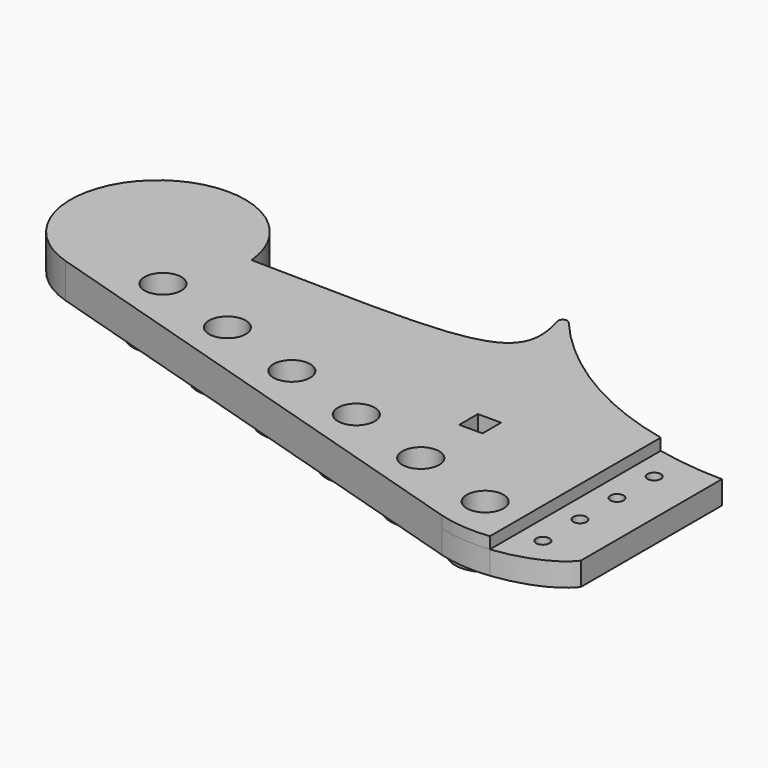
from build123d import *

# Parameters (mm, degrees)
F0_R      = 5.0419
F1_DEPTH  = 6.35
F2_DEPTH  = 9.525
F4_D      = 3.6576
F5_R      = 1.27
F8_W      = 6.35
F8_H      = 6.35
F9_DEPTH  = 9.5260001
F10_R     = 5.0419
F11_DEPTH = 3.175


with BuildPart() as f1:
    # F0 (on Top) → F1 (new body)
    with BuildSketch(Plane.XY):
        with BuildLine():
            Line((0, 0), (0, 24.13))
            ThreePointArc((0, 24.13), (-9.2620503813, 24.6926494565), (-18.415, 26.2176625565))
            Line((-18.415, 26.2176625565), (-18.415, -32.2023374435))
            add(Edge.make_bspline(
                [(-18.415, -32.2023374435), (-10.35310168, -31.3379440787), (-3.0120759205, -28.1461012273), (0, -24.13)],
                knots=[12.2106695442, 12.2106695442, 12.2106695442, 12.2106695442, 33.2224141479, 33.2224141479, 33.2224141479, 33.2224141479], degree=3))
            Line((0, -24.13), (0, 0))
        make_face()
        with BuildLine():
            Line((-18.415, -32.2023374435), (-18.415, 26.2176625565))
            ThreePointArc((-18.415, 26.2176625565), (-48.7549341061, 39.1874227389), (-72.2748938826, 62.3291118058))
            add(Edge.make_bspline(
                [(-137.9783539955, 35.7469866649), (-73.1067731977, 34.5293954015), (-59.7019699566, 33.2077455579), (-72.2748938826, 62.3291118058)],
                knots=[0, 0, 0, 0, 70.8770346997, 70.8770346997, 70.8770346997, 70.8770346997], degree=3))
            ThreePointArc((-137.9783539955, 35.7469866649), (-162.9147928474, 57.3381501066), (-185.674, 33.4629996115))
            ThreePointArc((-185.674, 33.4629996115), (-180.9856867862, 19.2452424177), (-168.7599080893, 10.6049162859))
            Line((-168.7599080893, 10.6049162859), (-32.4923986546, -31.0562422342))
            add(Edge.make_bspline(
                [(-32.4923986546, -31.0562422342), (-28.0285616621, -32.4209741599), (-23.1000548653, -32.7046670659), (-18.415, -32.2023374435)],
                knots=[0, 0, 0, 0, 12.2106695442, 12.2106695442, 12.2106695442, 12.2106695442], degree=3))
        make_face()
        with Locations((-99.2384759306, 1.0898536678)):
            Circle(F0_R, mode=Mode.SUBTRACT)
        with Locations((-122.5813012408, 8.226471557)):
            Circle(F0_R, mode=Mode.SUBTRACT)
        with Locations((-52.5528253102, -13.1833821107)):
            Circle(F0_R, mode=Mode.SUBTRACT)
        with Locations((-29.21, -20.32)):
            Circle(F0_R, mode=Mode.SUBTRACT)
        with Locations((-75.8956506204, -6.0467642215)):
            Circle(F0_R, mode=Mode.SUBTRACT)
        with Locations((-145.924126551, 15.3630894463)):
            Circle(F0_R, mode=Mode.SUBTRACT)
    extrude(amount=F1_DEPTH)

    # F0 (on Top) → F2 (join)
    with BuildSketch(Plane.XY):
        with BuildLine():
            Line((-18.415, -32.2023374435), (-18.415, 26.2176625565))
            ThreePointArc((-18.415, 26.2176625565), (-48.7549341061, 39.1874227389), (-72.2748938826, 62.3291118058))
            add(Edge.make_bspline(
                [(-137.9783539955, 35.7469866649), (-73.1067731977, 34.5293954015), (-59.7019699566, 33.2077455579), (-72.2748938826, 62.3291118058)],
                knots=[0, 0, 0, 0, 70.8770346997, 70.8770346997, 70.8770346997, 70.8770346997], degree=3))
            ThreePointArc((-137.9783539955, 35.7469866649), (-162.9147928474, 57.3381501066), (-185.674, 33.4629996115))
            ThreePointArc((-185.674, 33.4629996115), (-180.9856867862, 19.2452424177), (-168.7599080893, 10.6049162859))
            Line((-168.7599080893, 10.6049162859), (-32.4923986546, -31.0562422342))
            add(Edge.make_bspline(
                [(-32.4923986546, -31.0562422342), (-28.0285616621, -32.4209741599), (-23.1000548653, -32.7046670659), (-18.415, -32.2023374435)],
                knots=[0, 0, 0, 0, 12.2106695442, 12.2106695442, 12.2106695442, 12.2106695442], degree=3))
        make_face()
        with Locations((-99.2384759306, 1.0898536678)):
            Circle(F0_R, mode=Mode.SUBTRACT)
        with Locations((-122.5813012408, 8.226471557)):
            Circle(F0_R, mode=Mode.SUBTRACT)
        with Locations((-52.5528253102, -13.1833821107)):
            Circle(F0_R, mode=Mode.SUBTRACT)
        with Locations((-29.21, -20.32)):
            Circle(F0_R, mode=Mode.SUBTRACT)
        with Locations((-75.8956506204, -6.0467642215)):
            Circle(F0_R, mode=Mode.SUBTRACT)
        with Locations((-145.924126551, 15.3630894463)):
            Circle(F0_R, mode=Mode.SUBTRACT)
    extrude(amount=F2_DEPTH)

    # F4 (through all)
    with Locations(Plane.XY.offset(6.35)):
        with Locations((-12.065, 16.0576625565), (-12.065, 3.3576625565), (-12.065, -9.3423374435), (-12.065, -22.0423374435)):
            Hole(F4_D / 2)

    # F5
    f5_edges = [f1.edges().sort_by_distance(p)[0] for p in [
        (-72.274894, 62.329112, 3.175),
        (-72.274894, 62.329112, 7.9375),
    ]]
    fillet(f5_edges, radius=F5_R)

    # F8 (on Top) → F9 (cut, through all)
    with BuildSketch(Plane.XY):
        with Locations((-52.5528253102, 7.1366178893)):
            Rectangle(F8_W, F8_H)
    extrude(amount=F9_DEPTH, mode=Mode.SUBTRACT)

    # F10 (on face) → F11 (join)
    with BuildSketch(Plane(origin=(0, 0, 0), x_dir=(1, 0, 0), z_dir=(0, 0, -1))):
        with BuildLine():
            ThreePointArc((-29.21, 12.1031), (-23.3997742897, 14.5097742897), (-20.9931, 20.32))
            ThreePointArc((-20.9931, 20.32), (-29.21, 28.5369), (-37.4269, 20.32))
            ThreePointArc((-37.4269, 20.32), (-35.0202257103, 14.5097742897), (-29.21, 12.1031))
        make_face()
        with Locations((-29.21, 20.32)):
            Circle(F10_R, mode=Mode.SUBTRACT)
        with BuildLine():
            ThreePointArc((-29.21, 12.1031), (-35.0202257103, 14.5097742897), (-37.4269, 20.32))
            Line((-37.4269, 20.32), (-37.4269, 12.1031))
            Line((-37.4269, 12.1031), (-29.21, 12.1031))
        make_face()
        with BuildLine():
            ThreePointArc((-52.5528253102, 4.9664821107), (-58.3630510205, 7.3731564004), (-60.7697253102, 13.1833821107))
            Line((-60.7697253102, 13.1833821107), (-60.7697253102, 4.9664821107))
            Line((-60.7697253102, 4.9664821107), (-52.5528253102, 4.9664821107))
        make_face()
        with BuildLine():
            ThreePointArc((-44.3359253102, 13.1833821107), (-52.5528253102, 21.4002821107), (-60.7697253102, 13.1833821107))
            ThreePointArc((-60.7697253102, 13.1833821107), (-58.3630510205, 7.3731564004), (-52.5528253102, 4.9664821107))
            ThreePointArc((-52.5528253102, 4.9664821107), (-46.7425995999, 7.3731564004), (-44.3359253102, 13.1833821107))
        make_face()
        with Locations((-52.5528253102, 13.1833821107)):
            Circle(F10_R, mode=Mode.SUBTRACT)
        with BuildLine():
            ThreePointArc((-75.8956506204, -2.1701357785), (-81.7058763307, 0.2365385111), (-84.1125506204, 6.0467642215))
            Line((-84.1125506204, 6.0467642215), (-84.1125506204, -2.1701357785))
            Line((-84.1125506204, -2.1701357785), (-75.8956506204, -2.1701357785))
        make_face()
        with BuildLine():
            ThreePointArc((-67.6787506204, 6.0467642215), (-75.8956506204, 14.2636642215), (-84.1125506204, 6.0467642215))
            ThreePointArc((-84.1125506204, 6.0467642215), (-81.7058763307, 0.2365385111), (-75.8956506204, -2.1701357785))
            ThreePointArc((-75.8956506204, -2.1701357785), (-70.0854249101, 0.2365385111), (-67.6787506204, 6.0467642215))
        make_face()
        with Locations((-75.8956506204, 6.0467642215)):
            Circle(F10_R, mode=Mode.SUBTRACT)
        with BuildLine():
            ThreePointArc((-99.2384759306, -9.3067536678), (-105.0487016409, -6.9000793781), (-107.4553759306, -1.0898536678))
            Line((-107.4553759306, -1.0898536678), (-107.4553759306, -9.3067536678))
            Line((-107.4553759306, -9.3067536678), (-99.2384759306, -9.3067536678))
        make_face()
        with BuildLine():
            ThreePointArc((-91.0215759306, -1.0898536678), (-99.2384759306, 7.1270463322), (-107.4553759306, -1.0898536678))
            ThreePointArc((-107.4553759306, -1.0898536678), (-105.0487016409, -6.9000793781), (-99.2384759306, -9.3067536678))
            ThreePointArc((-99.2384759306, -9.3067536678), (-93.4282502203, -6.9000793781), (-91.0215759306, -1.0898536678))
        make_face()
        with Locations((-99.2384759306, -1.0898536678)):
            Circle(F10_R, mode=Mode.SUBTRACT)
        with BuildLine():
            ThreePointArc((-122.5813012408, -16.443371557), (-128.3915269511, -14.0366972674), (-130.7982012408, -8.226471557))
            Line((-130.7982012408, -8.226471557), (-130.7982012408, -16.443371557))
            Line((-130.7982012408, -16.443371557), (-122.5813012408, -16.443371557))
        make_face()
        with BuildLine():
            ThreePointArc((-114.3644012408, -8.226471557), (-122.5813012408, -0.009571557), (-130.7982012408, -8.226471557))
            ThreePointArc((-130.7982012408, -8.226471557), (-128.3915269511, -14.0366972674), (-122.5813012408, -16.443371557))
            ThreePointArc((-122.5813012408, -16.443371557), (-116.7710755305, -14.0366972674), (-114.3644012408, -8.226471557))
        make_face()
        with Locations((-122.5813012408, -8.226471557)):
            Circle(F10_R, mode=Mode.SUBTRACT)
        with BuildLine():
            ThreePointArc((-145.924126551, -23.5799894463), (-151.7343522614, -21.1733151566), (-154.141026551, -15.3630894463))
            Line((-154.141026551, -15.3630894463), (-154.141026551, -23.5799894463))
            Line((-154.141026551, -23.5799894463), (-145.924126551, -23.5799894463))
        make_face()
        with BuildLine():
            ThreePointArc((-137.707226551, -15.3630894463), (-145.924126551, -7.1461894463), (-154.141026551, -15.3630894463))
            ThreePointArc((-154.141026551, -15.3630894463), (-151.7343522614, -21.1733151566), (-145.924126551, -23.5799894463))
            ThreePointArc((-145.924126551, -23.5799894463), (-140.1139008407, -21.1733151566), (-137.707226551, -15.3630894463))
        make_face()
        with Locations((-145.924126551, -15.3630894463)):
            Circle(F10_R, mode=Mode.SUBTRACT)
    extrude(amount=F11_DEPTH)


solid = f1.part
